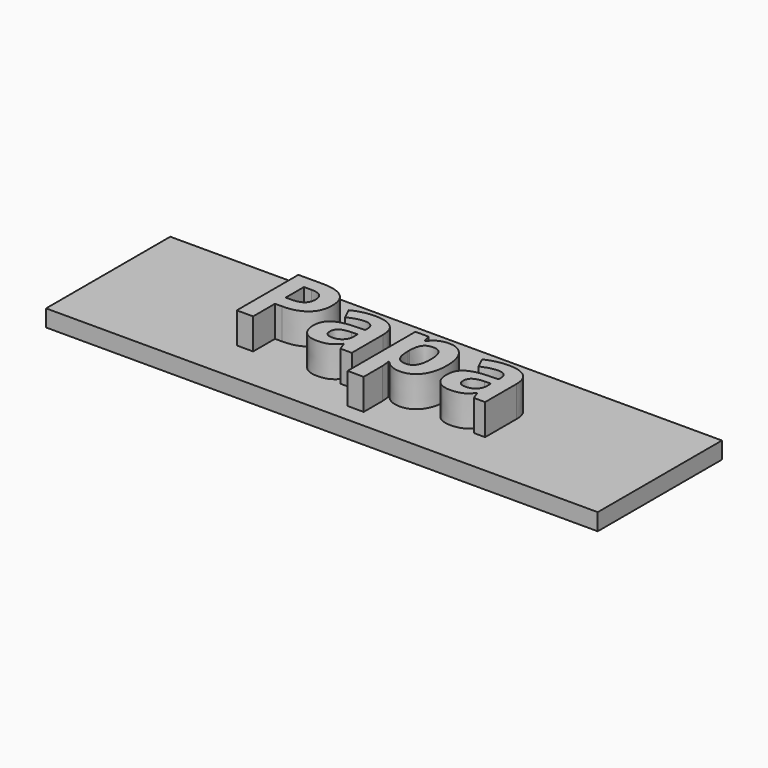
from build123d import *

# Parameters (mm, degrees)
F0_W         = 99.7281074524
F0_H         = 28.0603785068
F1_DEPTH     = 3.048
F2_TEXT_SIZE = 19.4863752565
F3_DEPTH     = 5.588


# Not quite as in the source:
# - Text() gives the source's letters only with a copy of the font that has no kerning and outlines rounded to 1/6400 em; it was checked with that copy


with BuildPart() as f1:
    # F0 (on Top) → F1 (new body)
    with BuildSketch(Plane.XY):
        Rectangle(F0_W, F0_H)
    extrude(amount=F1_DEPTH)

    # F2 (on face) → F3 (join)
    with BuildSketch(Plane.XY.offset(3.048)):
        with Locations((-23.5100468853, -6.0671095271)):
            Text('Papa', F2_TEXT_SIZE, font='Open Sans', font_style=FontStyle.BOLD, text_align=(TextAlign.LEFT, TextAlign.BOTTOM))
    extrude(amount=F3_DEPTH)


solid = f1.part
